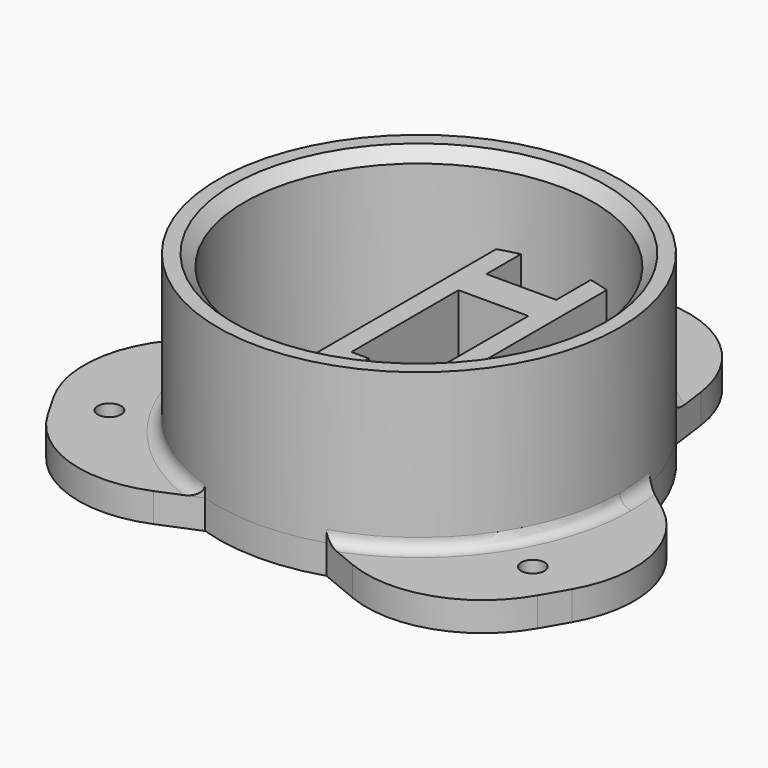
from build123d import *

# Parameters (mm, degrees)
F0_R         = 2
F0_R_2       = 30
F1_DEPTH     = 5
F2_R         = 34.5
F2_R_2       = 30
F3_DEPTH     = 27
F5_DEPTH     = 18
F6_SIZE      = 2
F7_T4_ANGLE  = 101.4429805126
F7_T10_ANGLE = 101.4429805126
F7_T16_ANGLE = 20.718590379
F7_T21_ANGLE = 80.7206862136
F8_W         = 6
F8_H         = 5
F9_DEPTH     = 10


# Not quite as in the source:
# - a fillet or chamfer that OpenCascade refuses, or shapes differently, is made with other operations: its cross-section is extruded or revolved along the edge and cut away or added


with BuildPart() as f1:
    # F0 (on Top) → F1 (new body)
    with BuildSketch(Plane.XY):
        with BuildLine():
            Line((2.4892725641, 50), (-2.4892725641, 50))
            ThreePointArc((-2.4892725641, 50), (-15.663935341, 45.0475333764), (-22.31389035, 32.6428260715))
            Line((-22.31389035, 32.6428260715), (-23.2700083459, 25.4707030052))
            ThreePointArc((-23.2700083459, 25.4707030052), (-29.8778764306, 17.25), (-33.6932800277, 7.4170668712))
            Line((-33.6932800277, 7.4170668712), (-39.4264618042, 3.0029828646))
            ThreePointArc((-39.4264618042, 3.0029828646), (-46.8442759523, -8.9584007597), (-44.5459064713, -22.8442267226))
            Line((-44.5459064713, -22.8442267226), (-42.0566339072, -27.1557732774))
            ThreePointArc((-42.0566339072, -27.1557732774), (-31.1803406113, -36.0891326167), (-17.1125714543, -35.6458089361))
            Line((-17.1125714543, -35.6458089361), (-10.4232716818, -32.8877698765))
            ThreePointArc((-10.4232716818, -32.8877698765), (0, -34.5), (10.4232716818, -32.8877698765))
            Line((10.4232716818, -32.8877698765), (17.1125714543, -35.6458089361))
            ThreePointArc((17.1125714543, -35.6458089361), (31.1803406113, -36.0891326167), (42.0566339072, -27.1557732774))
            Line((42.0566339072, -27.1557732774), (44.5459064713, -22.8442267226))
            ThreePointArc((44.5459064713, -22.8442267226), (46.8442759523, -8.9584007597), (39.4264618042, 3.0029828646))
            Line((39.4264618042, 3.0029828646), (33.6932800277, 7.4170668712))
            ThreePointArc((33.6932800277, 7.4170668712), (29.8778764306, 17.25), (23.2700083459, 25.4707030052))
            Line((23.2700083459, 25.4707030052), (22.31389035, 32.6428260715))
            ThreePointArc((22.31389035, 32.6428260715), (15.663935341, 45.0475333764), (2.4892725641, 50))
        make_face()
        with Locations((-36.3730669589, -21)):
            Circle(F0_R, mode=Mode.SUBTRACT)
        with Locations((36.3730669589, -21)):
            Circle(F0_R, mode=Mode.SUBTRACT)
        Circle(F0_R_2, mode=Mode.SUBTRACT)
        with Locations((0, 42)):
            Circle(F0_R, mode=Mode.SUBTRACT)
    extrude(amount=F1_DEPTH)

    # F2 (on face) → F3 (join)
    with BuildSketch(Plane.XY.offset(5)):
        Circle(F2_R)
        Circle(F2_R_2, mode=Mode.SUBTRACT)
    extrude(amount=F3_DEPTH)

    # F4 (on Top) → F5 (join)
    with BuildSketch(Plane.XY):
        with BuildLine():
            Line((9.5, 0), (9.5, 28.4561065503))
            ThreePointArc((9.5, 28.4561065503), (7.7641711286, 28.9778820255), (6, 29.3938769134))
            Line((6, 29.3938769134), (6, 22))
            Line((6, 22), (0, 22))
            Line((0, 22), (-6, 22))
            Line((-6, 22), (-6, 29.3938769134))
            ThreePointArc((-6, 29.3938769134), (-7.7641711286, 28.9778820255), (-9.5, 28.4561065503))
            Line((-9.5, 28.4561065503), (-9.5, 0))
            Line((-9.5, 0), (-9.5, -28.4561065503))
            ThreePointArc((-9.5, -28.4561065503), (-7.7641711286, -28.9778820255), (-6, -29.3938769134))
            Line((-6, -29.3938769134), (-6, -14))
            Line((-6, -14), (-6, -9))
            Line((-6, -9), (-6, -7))
            Line((-6, -7), (-6, 16))
            Line((-6, 16), (0, 16))
            Line((0, 16), (6, 16))
            Line((6, 16), (6, -7))
            Line((6, -7), (6, -9))
            Line((6, -9), (6, -14))
            Line((6, -14), (6, -29.3938769134))
            ThreePointArc((6, -29.3938769134), (7.7641711286, -28.9778820255), (9.5, -28.4561065503))
            Line((9.5, -28.4561065503), (9.5, 0))
        make_face()
        Polygon((0, -14), (6, -14), (6, -9), (6, -7), (3, -7), (3, -9), (-3, -9), (-3, -7), (-6, -7), (-6, -9), (-6, -14), align=None)
    extrude(amount=F5_DEPTH)

    # F6
    f6_edges = [f1.edges().sort_by_distance(p)[0] for p in [
        (-30, 0, 32),
    ]]
    chamfer(f6_edges, length=F6_SIZE)

    # F7: fillet of radius 2 on 3 edges, made by hand


with BuildPart() as f7_tool2:
    # F7_s3 → F7_t4 (revolve)
    with BuildSketch(Plane(origin=(0, 0, 0), x_dir=(0, 0, 1), z_dir=(0.3538256813, 0.9353113852, 0))):
        with BuildLine():
            ThreePointArc((7, -34.5), (5.5857864376, -35.0857864376), (5, -36.5))
            Line((5, -36.5), (5, -34.5))
            Line((5, -34.5), (7, -34.5))
        make_face()
    revolve(axis=Axis((0, 0, 5), (0, 0, 1)), revolution_arc=F7_T4_ANGLE)

    split(bisect_by=Plane(origin=(-16.1247319925, 20.9434209841, 0), x_dir=(0, 0, 1), z_dir=(0.6100531704, -0.7923604794, 0)), keep=Keep.TOP)

    split(bisect_by=Plane(origin=(10.0751686181, -24.4361380268, 0), x_dir=(0, 0, 1), z_dir=(-0.3811777189, 0.9245017829, 0)), keep=Keep.TOP)


with BuildPart() as f1_1:
    add(f1.part)

    # F7_t1: union F7_tool2
    add(f7_tool2.part)


with BuildPart() as f7_tool8:
    # F7_s9 → F7_t10 (revolve)
    with BuildSketch(Plane(origin=(0, 0, 0), x_dir=(0, 0, 1), z_dir=(0.6330905794, -0.7740777211, 0))):
        with BuildLine():
            ThreePointArc((7, -34.5), (5.5857864376, -35.0857864376), (5, -36.5))
            Line((5, -36.5), (5, -34.5))
            Line((5, -34.5), (7, -34.5))
        make_face()
    revolve(axis=Axis((0, 0, 5), (0, 0, 1)), revolution_arc=F7_T10_ANGLE)

    split(bisect_by=Plane(origin=(-26.1999006106, 3.4927170427, 0), x_dir=(0, 0, 1), z_dir=(0.9912308893, -0.1321413036, 0)), keep=Keep.TOP)

    split(bisect_by=Plane(origin=(26.1999006106, 3.4927170427, 0), x_dir=(0, 0, 1), z_dir=(-0.9912308893, -0.1321413036, 0)), keep=Keep.TOP)


with BuildPart() as f1_2:
    add(f1_1.part)

    # F7_t7: union F7_tool8
    add(f7_tool8.part)


with BuildPart() as f7_tool14:
    # F7_s15 → F7_t16 (revolve)
    with BuildSketch(Plane.XZ):
        with BuildLine():
            ThreePointArc((34.5, 7), (35.0857864376, 5.5857864376), (36.5, 5))
            Line((36.5, 5), (34.5, 5))
            Line((34.5, 5), (34.5, 7))
        make_face()
    revolve(axis=Axis((0, 0, 5), (0, 0, 1)), revolution_arc=F7_T16_ANGLE)

    split(bisect_by=Plane(origin=(16.1247319925, 20.9434209841, 0), x_dir=(0, 0, 1), z_dir=(-0.6100531704, -0.7923604794, 0)), keep=Keep.TOP)


with BuildPart() as f1_3:
    add(f1_2.part)

    # F7_t13: union F7_tool14
    add(f7_tool14.part)


with BuildPart() as f7_tool19:
    # F7_s20 → F7_t21 (revolve)
    with BuildSketch(Plane(origin=(0, 0, 0), x_dir=(0, 0, 1), z_dir=(-0.9869139979, -0.1612475137, 0))):
        with BuildLine():
            ThreePointArc((7, -34.5), (5.5857864376, -35.0857864376), (5, -36.5))
            Line((5, -36.5), (5, -34.5))
            Line((5, -34.5), (7, -34.5))
        make_face()
    revolve(axis=Axis((0, 0, 5), (0, 0, 1)), revolution_arc=F7_T21_ANGLE)

    split(bisect_by=Plane(origin=(-10.0751686181, -24.4361380268, 0), x_dir=(0, 0, 1), z_dir=(0.3811777189, 0.9245017829, 0)), keep=Keep.TOP)


with BuildPart() as f1_4:
    add(f1_3.part)

    # F7_t18: union F7_tool19
    add(f7_tool19.part)

    # F8 (on face) → F9 (cut)
    with BuildSketch(Plane(origin=(0, 0, 0), x_dir=(1, 0, 0), z_dir=(0, 0, -1))):
        with Locations((0, 11.5)):
            Rectangle(F8_W, F8_H)
    extrude(amount=-F9_DEPTH, mode=Mode.SUBTRACT)


solid = f1_4.part
